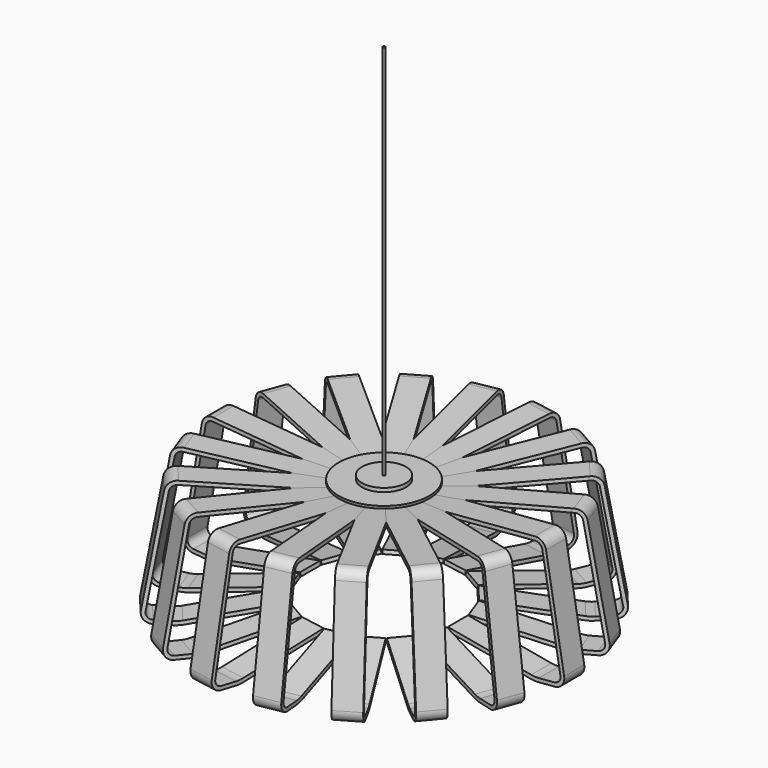
from build123d import *

# Parameters (mm, degrees)
F1_DEPTH = 20
F5_COUNT = 18
F5_ANGLE = 340


with BuildPart() as f1:
    # F0 (on Front) → F1 (new body, symmetric)
    with BuildSketch(Plane.XZ):
        with BuildLine():
            Line((64, 0), (60, 0))
            Line((60, 0), (60, -6))
            Line((60, -6), (72, -6))
            Line((72, -6), (256.8429673953, 9.4248201936))
            ThreePointArc((256.8429673953, 9.4248201936), (263.9596662181, 7.4032487391), (267.9767353142, 1.1905754693))
            Line((267.9767353142, 1.1905754693), (296.8251591927, -166.3438044046))
            ThreePointArc((296.8251591927, -166.3438044046), (295.0945778937, -174.9536302362), (287.4281021214, -179.2372223873))
            Line((287.4281021214, -179.2372223873), (262.5146952407, -181.3162023288))
            ThreePointArc((262.5146952407, -181.3162023288), (256.5120427189, -181.3260712694), (250.5514649721, -180.6165308408))
            Line((250.5514649721, -180.6165308408), (117.6975182293, -156.6409425299))
            Line((117.6975182293, -156.6409425299), (116.6260293193, -162.5444932848))
            Line((116.6260293193, -162.5444932848), (249.4799760621, -186.5200815957))
            ThreePointArc((249.4799760621, -186.5200815957), (256.4779613564, -187.2601308361), (263.5135067643, -187.1167018608))
            Line((263.5135067643, -187.1167018608), (288.426913645, -185.0377219193))
            ThreePointArc((288.426913645, -185.0377219193), (299.7651340841, -178.5447938861), (302.8272164841, -165.8429432908))
            Line((302.8272164841, -165.8429432908), (273.9787926057, 1.6914365831))
            ThreePointArc((273.9787926057, 1.6914365831), (267.6285138628, 12.1506863832), (255.8208984481, 15.3603849226))
            Line((255.8208984481, 15.3603849226), (71.461687531, -0.0240666446))
            Line((71.461687531, -0.0240666446), (65.4617357981, 0))
            Line((65.4617357981, 0), (65.2617357981, -2))
            Line((65.2617357981, -2), (63.6617357981, -2))
            Line((63.6617357981, -2), (64, 0))
        make_face()
    extrude(amount=F1_DEPTH, both=True)

    # F3 (on Front) → F4 (revolve)
    with BuildSketch(Plane.XZ):
        Polygon((35, -10), (72, -10), (72, -6.1), (59.9, -6.1), (59.9, 0.1), (64.15, 0.1), (64.3718317151, -1.8848128135), (65.6539957415, -1.8848128135), (65.85, 0.1), (72, 0.1), (72, 4), (35, 4), (35, 0), (25, 0), (25, -6), (35, -6), align=None)
    revolve(axis=Axis((0, 0, 2.3923777044), (0, 0, 1)))


with BuildPart() as f5_1:
    # F5: instance of F1
    add(f1.part.rotate(Axis((0, 0, 2.3923777044), (0, 0, 1)), 1 * F5_ANGLE / (F5_COUNT - 1)))


with BuildPart() as f5_2:
    # F5: instance of F1
    add(f1.part.rotate(Axis((0, 0, 2.3923777044), (0, 0, 1)), 2 * F5_ANGLE / (F5_COUNT - 1)))


with BuildPart() as f5_3:
    # F5: instance of F1
    add(f1.part.rotate(Axis((0, 0, 2.3923777044), (0, 0, 1)), 3 * F5_ANGLE / (F5_COUNT - 1)))


with BuildPart() as f5_4:
    # F5: instance of F1
    add(f1.part.rotate(Axis((0, 0, 2.3923777044), (0, 0, 1)), 4 * F5_ANGLE / (F5_COUNT - 1)))


with BuildPart() as f5_5:
    # F5: instance of F1
    add(f1.part.rotate(Axis((0, 0, 2.3923777044), (0, 0, 1)), 5 * F5_ANGLE / (F5_COUNT - 1)))


with BuildPart() as f5_6:
    # F5: instance of F1
    add(f1.part.rotate(Axis((0, 0, 2.3923777044), (0, 0, 1)), 6 * F5_ANGLE / (F5_COUNT - 1)))


with BuildPart() as f5_7:
    # F5: instance of F1
    add(f1.part.rotate(Axis((0, 0, 2.3923777044), (0, 0, 1)), 7 * F5_ANGLE / (F5_COUNT - 1)))


with BuildPart() as f5_8:
    # F5: instance of F1
    add(f1.part.rotate(Axis((0, 0, 2.3923777044), (0, 0, 1)), 8 * F5_ANGLE / (F5_COUNT - 1)))


with BuildPart() as f5_9:
    # F5: instance of F1
    add(f1.part.rotate(Axis((0, 0, 2.3923777044), (0, 0, 1)), 9 * F5_ANGLE / (F5_COUNT - 1)))


with BuildPart() as f5_10:
    # F5: instance of F1
    add(f1.part.rotate(Axis((0, 0, 2.3923777044), (0, 0, 1)), 10 * F5_ANGLE / (F5_COUNT - 1)))


with BuildPart() as f5_11:
    # F5: instance of F1
    add(f1.part.rotate(Axis((0, 0, 2.3923777044), (0, 0, 1)), 11 * F5_ANGLE / (F5_COUNT - 1)))


with BuildPart() as f5_12:
    # F5: instance of F1
    add(f1.part.rotate(Axis((0, 0, 2.3923777044), (0, 0, 1)), 12 * F5_ANGLE / (F5_COUNT - 1)))


with BuildPart() as f5_13:
    # F5: instance of F1
    add(f1.part.rotate(Axis((0, 0, 2.3923777044), (0, 0, 1)), 13 * F5_ANGLE / (F5_COUNT - 1)))


with BuildPart() as f5_14:
    # F5: instance of F1
    add(f1.part.rotate(Axis((0, 0, 2.3923777044), (0, 0, 1)), 14 * F5_ANGLE / (F5_COUNT - 1)))


with BuildPart() as f5_15:
    # F5: instance of F1
    add(f1.part.rotate(Axis((0, 0, 2.3923777044), (0, 0, 1)), 15 * F5_ANGLE / (F5_COUNT - 1)))


with BuildPart() as f5_16:
    # F5: instance of F1
    add(f1.part.rotate(Axis((0, 0, 2.3923777044), (0, 0, 1)), 16 * F5_ANGLE / (F5_COUNT - 1)))


with BuildPart() as f5_17:
    # F5: instance of F1
    add(f1.part.rotate(Axis((0, 0, 2.3923777044), (0, 0, 1)), 17 * F5_ANGLE / (F5_COUNT - 1)))


with BuildPart() as f8:
    # F6 (on Front) → F8 (revolve)
    with BuildSketch(Plane.XZ):
        Polygon((0, 610), (0, 0), (35, 0), (35, 10), (2, 10), (2, 610), align=None)
    revolve(axis=Axis((0, 0, 315.4409773648), (0, 0, 1)))


solid = Compound([f1.part, f5_1.part, f5_2.part, f5_3.part, f5_4.part, f5_5.part, f5_6.part, f5_7.part, f5_8.part, f5_9.part, f5_10.part, f5_11.part, f5_12.part, f5_13.part, f5_14.part, f5_15.part, f5_16.part, f5_17.part, f8.part])
